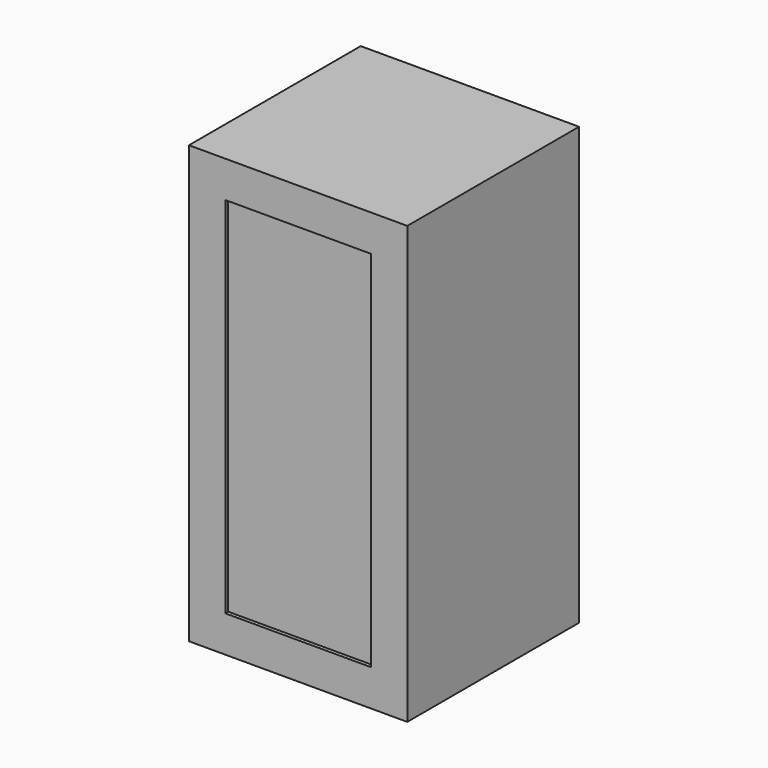
from build123d import *

# Parameters (mm, degrees)
F0_W     = 381
F0_H     = 762
F0_W_2   = 254
F0_H_2   = 635
F1_DEPTH = 374.65
F2_DEPTH = 6.35


# Not quite as in the source:
# - a feature names something its author has since deleted; it is built from what else it names


with BuildPart() as f1:
    # F0 (on Front) → F1 (new body)
    with BuildSketch(Plane.XZ):
        with Locations((73.4267770052, 381)):
            Rectangle(F0_W, F0_H)
        with Locations((73.4267770052, 381)):
            Rectangle(F0_W_2, F0_H_2, mode=Mode.SUBTRACT)
        with Locations((73.4267770052, 381)):
            Rectangle(F0_W_2, F0_H_2)
    extrude(amount=-F1_DEPTH)

    # F0 (on Front) → F2 (cut)
    with BuildSketch(Plane.XZ):
        with Locations((73.4267770052, 381)):
            Rectangle(F0_W_2, F0_H_2)
    extrude(amount=-F2_DEPTH, mode=Mode.SUBTRACT)


solid = f1.part
